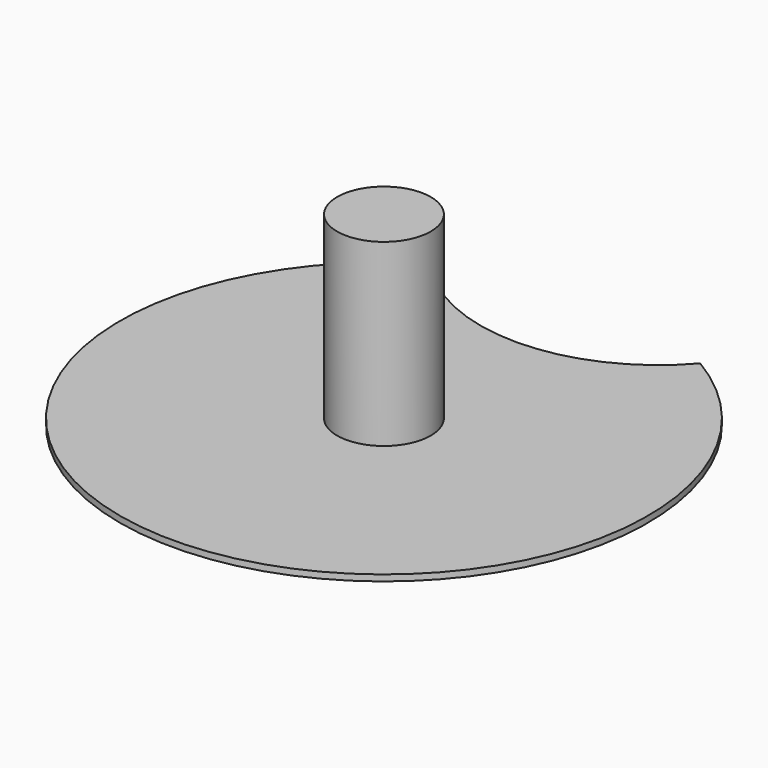
from build123d import *

# Parameters (mm, degrees)
F0_R     = 54.0947036541
F1_DEPTH = 1.27
F2_R     = 36.4799484266
F3_DEPTH = 25.4
F4_R     = 9.5951765944
F5_DEPTH = 38.1


# Not quite as in the source:
# - the program builds the solid bodies; features that only make, move or delete a surface that nothing else refers to are left out


with BuildPart() as f1:
    # F0 (on Top) → F1 (new body)
    with BuildSketch(Plane.XY):
        Circle(F0_R)
    extrude(amount=F1_DEPTH)

    # F2 (on Top) → F3 (cut)
    with BuildSketch(Plane.XY):
        with Locations((0, 70.3405514359)):
            Circle(F2_R)
    extrude(amount=F3_DEPTH, mode=Mode.SUBTRACT)

    # F4 (on Top) → F5 (join)
    with BuildSketch(Plane.XY):
        Circle(F4_R)
    extrude(amount=F5_DEPTH)


solid = f1.part
